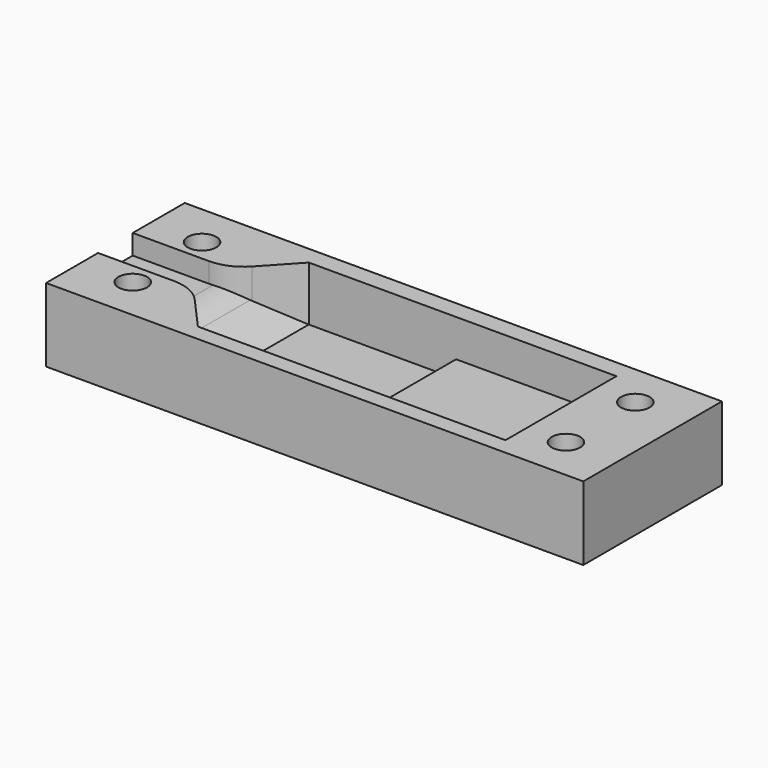
from build123d import *

# Parameters (mm, degrees)
F0_W         = 65
F0_H         = 20
F1_DEPTH     = 7.5
F3_DEPTH     = 2.5
F4_R         = 1.65
F5_DEPTH     = 5
F7_DEPTH     = 3.3
F8_W         = 12
F8_H         = 16
F9_DEPTH     = 2
F10_R        = 1.35
F11_DEPTH    = 5
F12_T4_DEPTH = 16
F15_DEPTH    = 2
F16_DEPTH    = 20
F17_W        = 20
F17_H        = 7.5
F18_DEPTH    = 3
F19_W        = 10.9964999743
F19_H        = 5
F20_DEPTH    = 2
F21_DEPTH    = 1
F22_R        = 5
F23_DEPTH    = 0.5


# Not quite as in the source:
# - a fillet or chamfer that OpenCascade refuses, or shapes differently, is made with other operations: its cross-section is extruded or revolved along the edge and cut away or added


with BuildPart() as f1:
    # F0 (on Top) → F1 (new body)
    with BuildSketch(Plane.XY):
        with Locations((32.5, 10)):
            Rectangle(F0_W, F0_H)
    extrude(amount=F1_DEPTH)

    # F2 (on face) → F3 (cut)
    with BuildSketch(Plane(origin=(0, 0, 0), x_dir=(1, 0, 0), z_dir=(0, 0, -1))):
        Polygon((4.375, -7.8145825623), (7.625, -7.8145825623), (9.25, -5), (7.625, -2.1854174377), (4.375, -2.1854174377), (2.75, -5), align=None)
        Polygon((7.625, -12.1854174377), (4.375, -12.1854174377), (2.75, -15), (4.375, -17.8145825623), (7.625, -17.8145825623), (9.25, -15), align=None)
        Polygon((54.375, -7.8145825623), (57.625, -7.8145825623), (59.25, -5), (57.625, -2.1854174377), (54.375, -2.1854174377), (52.75, -5), align=None)
        Polygon((54.375, -17.8145825623), (57.625, -17.8145825623), (59.25, -15), (57.625, -12.1854174377), (54.375, -12.1854174377), (52.75, -15), align=None)
    extrude(amount=-F3_DEPTH, mode=Mode.SUBTRACT)

    # F4 (on face) → F5 (cut)
    with BuildSketch(Plane(origin=(0, 0, 2.5), x_dir=(1, 0, 0), z_dir=(0, 0, -1))):
        with Locations((6, -5)):
            Circle(F4_R)
        with Locations((6, -15)):
            Circle(F4_R)
        with Locations((56, -5)):
            Circle(F4_R)
        with Locations((56, -15)):
            Circle(F4_R)
    extrude(amount=-F5_DEPTH, mode=Mode.SUBTRACT)

    # F6 (on face) → F7 (cut)
    with BuildSketch(Plane.XY.offset(7.5)):
        Polygon((51, 17.9014432635), (16, 17.9014432635), (16, 12.5), (16, 7.5), (16, 1.9014432635), (51, 1.9014432635), align=None)
        Polygon((16, 12.5), (16, 17.9014432635), (11, 12.5), align=None)
        Polygon((16, 7.5), (16, 12.5), (11, 12.5), (0, 12.5), (0, 7.5), (11, 7.5), align=None)
        Polygon((16, 1.9014432635), (16, 7.5), (11, 7.5), align=None)
    extrude(amount=-F7_DEPTH, mode=Mode.SUBTRACT)

    # F8 (on face) → F9 (cut)
    with BuildSketch(Plane.XY.offset(4.2)):
        with Locations((22, 9.9014432635)):
            Rectangle(F8_W, F8_H)
    extrude(amount=-F9_DEPTH, mode=Mode.SUBTRACT)

    # F10 (on face) → F11 (cut)
    with BuildSketch(Plane.XY.offset(4.2)):
        with Locations((47.8, 14.9014432635)):
            Circle(F10_R)
        with Locations((47.8, 4.9014432635)):
            Circle(F10_R)
    extrude(amount=-F11_DEPTH, mode=Mode.SUBTRACT)

    # F12: chamfer of 5 on 1 edges, made by hand


with BuildPart() as f12_tool2:
    # F12_s3 → F12_t4 (new body)
    with BuildSketch(Plane.XZ.offset(-1.9014432635)):
        Polygon((33, 4.2), (28, -0.8), (28, 4.2), align=None)
    extrude(amount=-F12_T4_DEPTH)

    split(bisect_by=Plane.XY.offset(2.2), keep=Keep.TOP)


with BuildPart() as f1_1:
    add(f1.part)

    # F12_t1: cut F12_tool2
    add(f12_tool2.part, mode=Mode.SUBTRACT)

    # F14 (on face) → F15 (cut)
    with BuildSketch(Plane.XY.offset(4.2)):
        Polygon((16, 17.9014432635), (11, 12.5), (11, 7.5), (16, 1.9014432635), align=None)
    extrude(amount=-F15_DEPTH, mode=Mode.SUBTRACT)

    # F13 (on face) → F16 (join)
    with BuildSketch(Plane.XZ):
        Polygon((10.9964999743, 2.2), (15.9964999743, 2.2), (10.9964999743, 6.2), align=None)
    extrude(amount=-F16_DEPTH)

    # F17 (on face) → F18 (cut)
    with BuildSketch(Plane.YZ.offset(65)):
        with Locations((10, 3.75)):
            Rectangle(F17_W, F17_H)
    extrude(amount=-F18_DEPTH, mode=Mode.SUBTRACT)

    # F19 (on face) → F20 (join)
    with BuildSketch(Plane.XY.offset(4.2)):
        with Locations((5.4982499871, 10)):
            Rectangle(F19_W, F19_H)
    extrude(amount=F20_DEPTH)

    # F21 (add): a face of the model
    f21_faces = [f1_1.faces().sort_by_distance(p)[0] for p in [
        (61.348540101, 10, 7.5),
    ]]
    extrude(f21_faces, amount=F21_DEPTH)

    # F22 (call 1 of 3: OpenCascade refuses the feature's edges together)
    f22_edges = [f1_1.edges().sort_by_distance(p)[0] for p in [
        (11, 12.5, 7.3486),
    ]]
    fillet(f22_edges, radius=F22_R)

    # F22#2 (call 2 of 3)
    f22_2_edges = [f1_1.edges().sort_by_distance(p)[0] for p in [
        (10.9965, 10, 6.2),
    ]]
    fillet(f22_2_edges, radius=F22_R)

    # F22#3 (call 3 of 3)
    f22_3_edges = [f1_1.edges().sort_by_distance(p)[0] for p in [
        (11, 7.5, 7.3486),
    ]]
    fillet(f22_3_edges, radius=F22_R)

    # F23 (cut): a face of the model
    f23_faces = [f1_1.faces().sort_by_distance(p)[0] for p in [
        (51, 9.9014432635, 6.35),
    ]]
    extrude(f23_faces, amount=-F23_DEPTH, mode=Mode.SUBTRACT)


solid = f1_1.part
